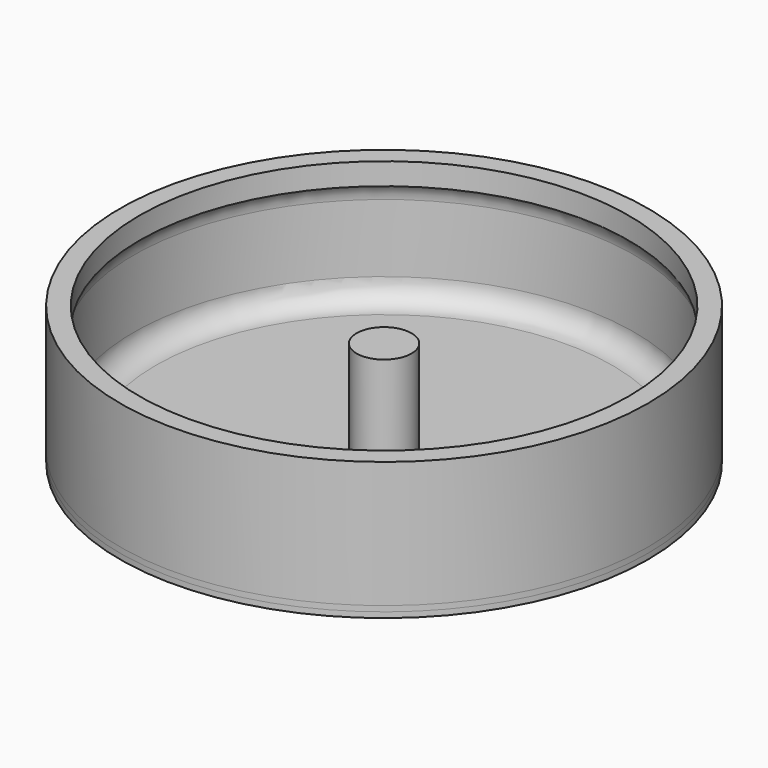
from build123d import *

# Parameters (mm, degrees)
F0_R     = 24
F1_DEPTH = 12
F2_R     = 22.25
F3_DEPTH = 13
F5_R     = 22.75
F6_DEPTH = 10
F4_R     = 2.5
F7_DEPTH = 9
F8_R     = 24
F9_DEPTH = 0.5


# Not quite as in the source:
# - a fillet or chamfer that OpenCascade refuses, or shapes differently, is made with other operations: its cross-section is extruded or revolved along the edge and cut away or added


with BuildPart() as f1:
    # F0 (on Top) → F1 (new body)
    with BuildSketch(Plane.XY):
        Circle(F0_R)
    extrude(amount=F1_DEPTH)

    # F2 (on Top) → F3 (cut)
    with BuildSketch(Plane.XY):
        Circle(F2_R)
    extrude(amount=F3_DEPTH, mode=Mode.SUBTRACT)

    # F5 (on Top) → F6 (cut)
    with BuildSketch(Plane.XY):
        Circle(F5_R)
    extrude(amount=F6_DEPTH, mode=Mode.SUBTRACT)



with BuildPart() as f7:
    # F4 (on Top) → F7 (new body)
    with BuildSketch(Plane.XY):
        Circle(F4_R)
    extrude(amount=F7_DEPTH)


with BuildPart() as f1_1:
    add(f1.part)

    add(f7.part)  # F9 merges F7
    # F8 (on Top) → F9 (join, symmetric)
    with BuildSketch(Plane.XY):
        Circle(F8_R)
    extrude(amount=F9_DEPTH, both=True)

    # F10: fillet of radius 2 on 3 edges, made by hand

    # F10_s1 → F10_t2 (revolve)
    with BuildSketch(Plane.XZ):
        with BuildLine():
            ThreePointArc((20.75, 0.5), (22.1642135624, 1.0857864376), (22.75, 2.5))
            Line((22.75, 2.5), (22.75, 0.5))
            Line((22.75, 0.5), (20.75, 0.5))
        make_face()
    revolve(axis=Axis((0, 0, 0.5), (0, 0, -1)))

    # F10_s3 → F10_t4 (revolve)
    with BuildSketch(Plane.XZ):
        with BuildLine():
            ThreePointArc((22.75, 8.6771243445), (22.6208286934, 9.3842311257), (22.25, 10))
            Line((22.25, 10), (22.75, 10))
            Line((22.75, 10), (22.75, 8.6771243445))
        make_face()
    revolve(axis=Axis((0, 0, 10), (0, 0, 1)))


solid = f1_1.part
